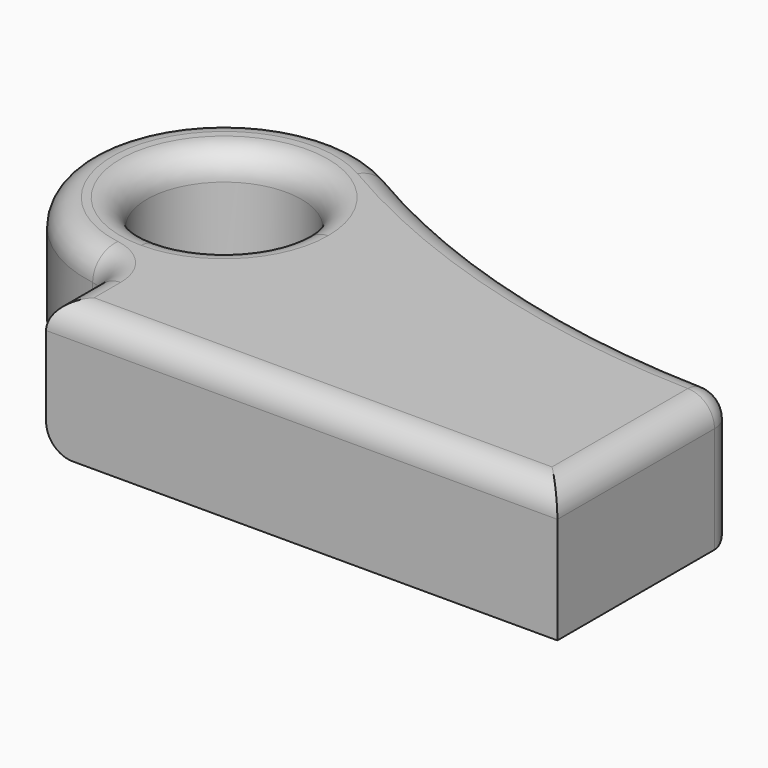
from build123d import *

# Parameters (mm, degrees)
F1_DEPTH = 25
F3_R     = 5


# Not quite as in the source:
# - the program builds the solid bodies; features that only make, move or delete a surface that nothing else refers to are left out


with BuildPart() as f1:
    # F0 (on Top) → F1 (new body)
    with BuildSketch(Plane.XY):
        with BuildLine():
            Line((-22.0192338504, 20.8813082427), (47.958523035, 20.8813082427))
            ThreePointArc((47.958523035, 20.8813082427), (5.048852146, 26.5810643591), (-34.884897805, 43.2850366545))
            ThreePointArc((-34.884897805, 43.2850366545), (-25.4644430478, 33.7988578917), (-22.0192338504, 20.8813082427))
        make_face()
        with BuildLine():
            ThreePointArc((-34.884897805, 43.2850366545), (-72.9983264837, 27.652937785), (-47.958523035, -5.057980942))
            Line((-47.958523035, -5.057980942), (-47.958523035, 6.3973983269))
            ThreePointArc((-47.958523035, 6.3973983269), (-58.2001939546, 31.1229791622), (-33.4746131192, 20.8813082427))
            Line((-33.4746131192, 20.8813082427), (-22.0192338504, 20.8813082427))
            ThreePointArc((-22.0192338504, 20.8813082427), (-25.4644430478, 33.7988578917), (-34.884897805, 43.2850366545))
        make_face()
        with BuildLine():
            Line((-47.958523035, 6.3973983269), (-47.958523035, -5.057980942))
            ThreePointArc((-47.958523035, -5.057980942), (-29.6166757534, 2.539460961), (-22.0192338504, 20.8813082427))
            Line((-22.0192338504, 20.8813082427), (-33.4746131192, 20.8813082427))
            ThreePointArc((-33.4746131192, 20.8813082427), (-37.7168521155, 10.6396373231), (-47.958523035, 6.3973983269))
        make_face()
        with BuildLine():
            Line((-47.958523035, -5.057980942), (-47.958523035, -20.8813082427))
            Line((-47.958523035, -20.8813082427), (47.958523035, -20.8813082427))
            Line((47.958523035, -20.8813082427), (47.958523035, 20.8813082427))
            Line((47.958523035, 20.8813082427), (-22.0192338504, 20.8813082427))
            ThreePointArc((-22.0192338504, 20.8813082427), (-29.6166757534, 2.539460961), (-47.958523035, -5.057980942))
        make_face()
    extrude(amount=-F1_DEPTH)

    # F3
    f3_edges = [f1.edges().sort_by_distance(p)[0] for p in [
        (5.048852, 26.581064, 0),
        (-72.998326, 27.652938, 0),
        (-47.958523, -12.969645, 0),
        (0, -20.881308, 0),
        (47.958523, 0, 0),
        (-62.442433, 20.881308, 0),
        (47.958523, 20.881308, -12.5),
        (-34.884898, 43.285037, -12.5),
        (5.048852, 26.581064, -25),
        (-47.958523, -5.057981, -12.5),
        (-72.998326, 27.652938, -25),
        (-47.958523, -12.969645, -25),
    ]]
    fillet(f3_edges, radius=F3_R)


solid = f1.part
